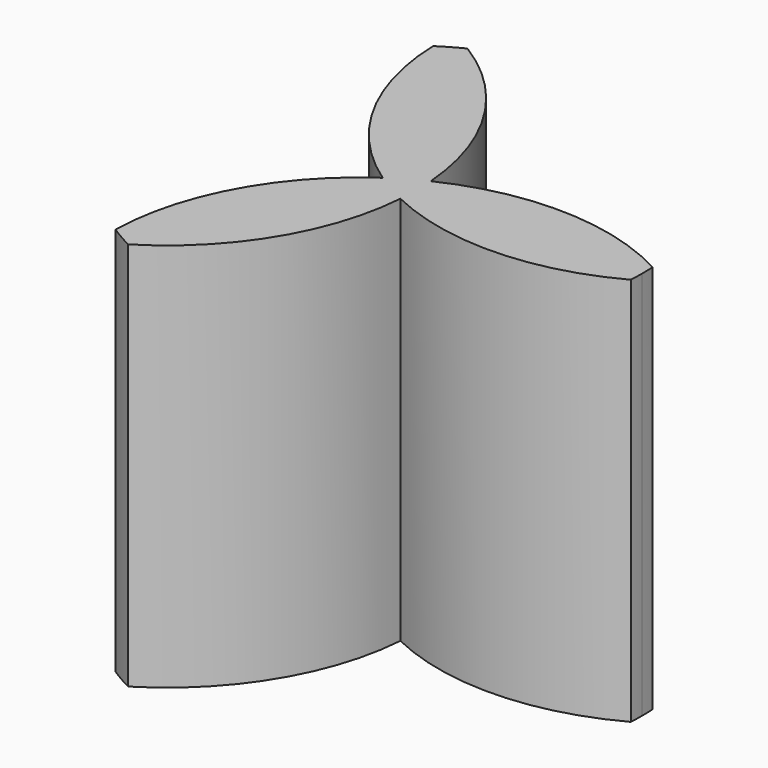
from build123d import *

# Parameters (mm, degrees)
F1_DEPTH = 5


with BuildPart() as f1:
    # F0 (on Top) → F1 (new body)
    with BuildSketch(Plane.XY):
        with BuildLine():
            ThreePointArc((3.0449996355, -0.1745772603), (3.0487496526, -0.0873244288), (3.05, 0))
            ThreePointArc((3.05, 0), (3.0487496526, 0.0873244288), (3.0449996355, 0.1745772603))
            ThreePointArc((3.0449996355, 0.1745772603), (1.6011501733, 0.55771632), (0.140706095, 0.2437101054))
            ThreePointArc((0.140706095, 0.2437101054), (0.1476756796, 0.1219436265), (0.15, 0))
            ThreePointArc((0.15, 0), (0.1476756796, -0.1219436265), (0.140706095, -0.2437101054))
            ThreePointArc((0.140706095, -0.2437101054), (1.6011501733, -0.55771632), (3.0449996355, -0.1745772603))
        make_face()
        with BuildLine():
            ThreePointArc((0.140706095, 0.2437101054), (-0.3175785854, 1.6654948853), (-1.3713114754, 2.724335669))
            ThreePointArc((-1.3713114754, 2.724335669), (-1.525, 2.6413774815), (-1.6736881601, 2.5497584087))
            ThreePointArc((-1.6736881601, 2.5497584087), (-1.2835715879, 1.1077785653), (-0.28141219, 0))
            ThreePointArc((-0.28141219, 0), (-0.075, 0.1299038106), (0.140706095, 0.2437101054))
        make_face()
        with BuildLine():
            ThreePointArc((0.15, 0), (0.1476756796, 0.1219436265), (0.140706095, 0.2437101054))
            ThreePointArc((0.140706095, 0.2437101054), (-0.075, 0.1299038106), (-0.28141219, 0))
            ThreePointArc((-0.28141219, 0), (-0.075, -0.1299038106), (0.140706095, -0.2437101054))
            ThreePointArc((0.140706095, -0.2437101054), (0.1476756796, -0.1219436265), (0.15, 0))
        make_face()
        with BuildLine():
            ThreePointArc((-1.6736881601, -2.5497584087), (-1.525, -2.6413774815), (-1.3713114754, -2.724335669))
            ThreePointArc((-1.3713114754, -2.724335669), (-0.3175785854, -1.6654948853), (0.140706095, -0.2437101054))
            ThreePointArc((0.140706095, -0.2437101054), (-0.075, -0.1299038106), (-0.28141219, 0))
            ThreePointArc((-0.28141219, 0), (-1.2835715879, -1.1077785653), (-1.6736881601, -2.5497584087))
        make_face()
    extrude(amount=F1_DEPTH)


solid = f1.part
